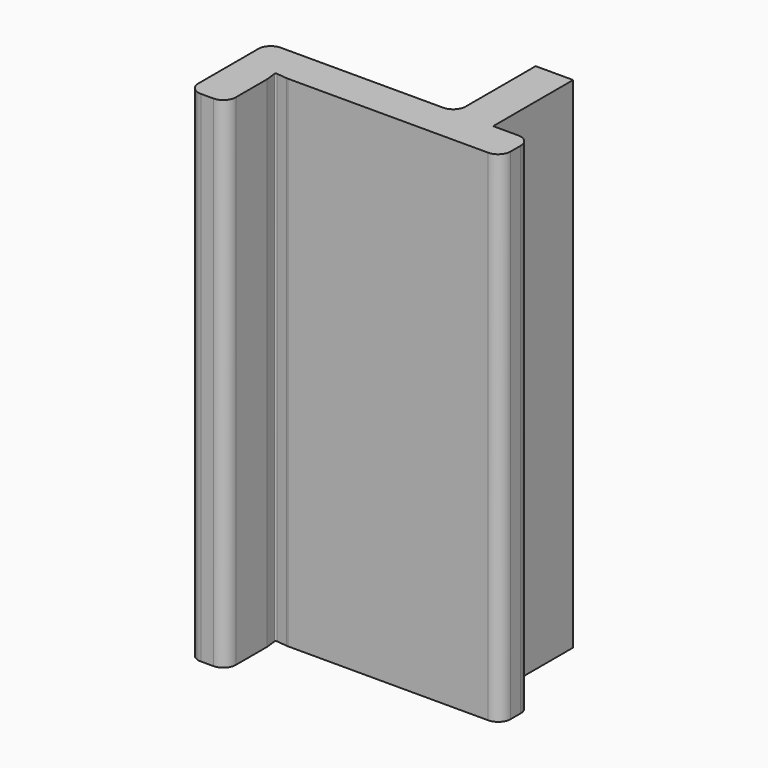
from build123d import *

# Parameters (mm, degrees)
F0_W     = 3
F0_H     = 8
F0_H_2   = 3
F1_DEPTH = 40
F2_R     = 1


with BuildPart() as f1:
    # F0 (on Top) → F1 (new body)
    with BuildSketch(Plane.XY):
        with BuildLine():
            Line((-14.0882119191, 0), (0, 0))
            Line((0, 0), (0, 3))
            Line((0, 3), (-3, 3))
            Line((-3, 3), (-18, 3))
            Line((-18, 3), (-18, -5))
            Line((-18, -5), (-15, -5))
            Line((-15, -5), (-15, -0.87328878))
            Line((-15, -0.87328878), (-15.0993422135, -0.0114509659))
            ThreePointArc((-15.0993422135, -0.0114509659), (-15.0708824979, 0.0705384398), (-14.9890325392, 0.0993967545))
            Line((-14.9890325392, 0.0993967545), (-14.0882119191, 0))
        make_face()
        with Locations((-1.5, 7)):
            Rectangle(F0_W, F0_H)
        with Locations((1.5, 1.5)):
            Rectangle(F0_W, F0_H_2)
    extrude(amount=F1_DEPTH)

    # F2
    f2_edges = [f1.edges().sort_by_distance(p)[0] for p in [
        (-18, -5, 20),
        (-15, -5, 20),
        (-18, 3, 20),
        (3, 0, 20),
        (3, 3, 20),
        (-3, 3, 20),
        (-14.088212, 0, 20),
    ]]
    fillet(f2_edges, radius=F2_R)


solid = f1.part
